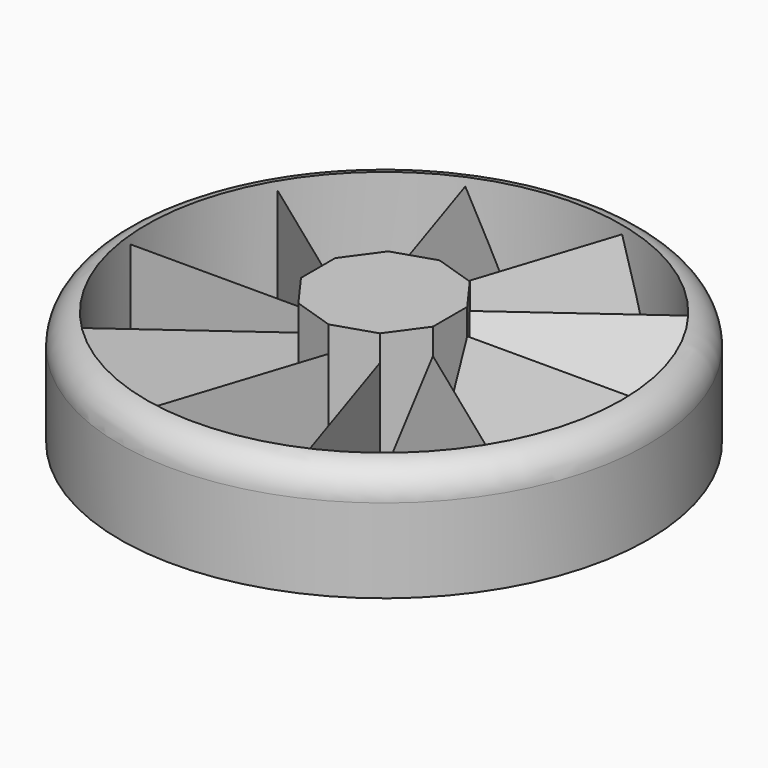
from build123d import *

# Parameters (mm, degrees)
F1_DEPTH  = 15
F3_DEPTH  = 20
F5_DEPTH  = 20
F14_DEPTH = 20
F15_DEPTH = 20
F16_DEPTH = 20
F17_DEPTH = 20
F18_DEPTH = 20
F19_DEPTH = 20
F20_DEPTH = 20
F21_DEPTH = 20
F23_R     = 30
F23_R_2   = 27
F24_DEPTH = 13
F26_R     = 1
F27_DEPTH = 8


# Not quite as in the source:
# - a fillet or chamfer that OpenCascade refuses, or shapes differently, is made with other operations: its cross-section is extruded or revolved along the edge and cut away or added


with BuildPart() as f1:
    # F0 (on Top) → F1 (new body)
    with BuildSketch(Plane.XY):
        Polygon((7.5, -2.4368977217), (7.5, 2.4368977217), (4.6352549156, 6.3798810626), (0, 7.8859666818), (-4.6352549156, 6.3798810626), (-7.5, 2.4368977217), (-7.5, -2.4368977217), (-4.6352549156, -6.3798810626), (0, -7.8859666818), (4.6352549156, -6.3798810626), align=None)
    extrude(amount=F1_DEPTH)

    # F2 (on face) → F3 (join)
    with BuildSketch(Plane(origin=(-2.3176274578, -7.1329238722, 0), x_dir=(0.9510565163, -0.3090169944, 0), z_dir=(-0.3090169944, -0.9510565163, 0))):
        Polygon((2.4368977217, 12.0518097386), (-2.4368977217, 0), (2.4368977217, 0), align=None)
    extrude(amount=F3_DEPTH)

    # F4 (on face) → F5 (join)
    with BuildSketch(Plane(origin=(-6.0676274578, -4.4083893922, 0), x_dir=(0.5877852523, -0.8090169944, 0), z_dir=(-0.8090169944, -0.5877852523, 0))):
        Polygon((2.4368977217, 12.0518097386), (-2.4368977217, 0), (2.4368977217, 0), align=None)
    extrude(amount=F5_DEPTH)

    # F13 (on face) → F14 (join)
    with BuildSketch(Plane(origin=(2.3176274578, -7.1329238722, 0), x_dir=(0.9510565163, 0.3090169944, 0), z_dir=(0.3090169944, -0.9510565163, 0))):
        Polygon((2.4368977217, 12.0518097386), (-2.4368977217, 0), (2.4368977217, 0), align=None)
    extrude(amount=F14_DEPTH)

    # F12 (on face) → F15 (join)
    with BuildSketch(Plane(origin=(6.0676274578, -4.4083893922, 0), x_dir=(0.5877852523, 0.8090169944, 0), z_dir=(0.8090169944, -0.5877852523, 0))):
        Polygon((2.4368977217, 12.0518097386), (-2.4368977217, 0), (2.4368977217, 0), align=None)
    extrude(amount=F15_DEPTH)

    # F11 (on face) → F16 (join)
    with BuildSketch(Plane.YZ.offset(7.5)):
        Polygon((2.4368977217, 12.0518097386), (-2.4368977217, 0), (2.4368977217, 0), align=None)
    extrude(amount=F16_DEPTH)

    # F10 (on face) → F17 (join)
    with BuildSketch(Plane(origin=(6.0676274578, 4.4083893922, 0), x_dir=(-0.5877852523, 0.8090169944, 0), z_dir=(0.8090169944, 0.5877852523, 0))):
        Polygon((2.4368977217, 12.0518097386), (-2.4368977217, 0), (2.4368977217, 0), align=None)
    extrude(amount=F17_DEPTH)

    # F9 (on face) → F18 (join)
    with BuildSketch(Plane(origin=(2.3176274578, 7.1329238722, 0), x_dir=(-0.9510565163, 0.3090169944, 0), z_dir=(0.3090169944, 0.9510565163, 0))):
        Polygon((2.4368977217, 12.0518097386), (-2.4368977217, 0), (2.4368977217, 0), align=None)
    extrude(amount=F18_DEPTH)

    # F8 (on face) → F19 (join)
    with BuildSketch(Plane(origin=(-2.3176274578, 7.1329238722, 0), x_dir=(-0.9510565163, -0.3090169944, 0), z_dir=(-0.3090169944, 0.9510565163, 0))):
        Polygon((2.4368977217, 12.0518097386), (-2.4368977217, 0), (2.4368977217, 0), align=None)
    extrude(amount=F19_DEPTH)

    # F7 (on face) → F20 (join)
    with BuildSketch(Plane(origin=(-6.0676274578, 4.4083893922, 0), x_dir=(-0.5877852523, -0.8090169944, 0), z_dir=(-0.8090169944, 0.5877852523, 0))):
        Polygon((2.4368977217, 12.0518097386), (-2.4368977217, 0), (2.4368977217, 0), align=None)
    extrude(amount=F20_DEPTH)

    # F6 (on face) → F21 (join)
    with BuildSketch(Plane(origin=(-7.5, 0, 0), x_dir=(0, -1, 0), z_dir=(-1, 0, 0))):
        Polygon((2.4368977217, 12.0518097386), (-2.4368977217, 0), (2.4368977217, 0), align=None)
    extrude(amount=F21_DEPTH)

    # F23 (on face) → F24 (join)
    with BuildSketch(Plane.XY):
        Circle(F23_R)
        Circle(F23_R_2, mode=Mode.SUBTRACT)
    extrude(amount=F24_DEPTH)

    # F25: fillet of radius 3.5 on 1 edges, made by hand

    # F25_s1 → F25_t2 (revolve, cut)
    with BuildSketch(Plane.XZ):
        with BuildLine():
            ThreePointArc((27, 13), (29.1457513111, 11.8271862323), (30, 9.5358983849))
            Line((30, 9.5358983849), (30, 13))
            Line((30, 13), (27, 13))
        make_face()
    revolve(axis=Axis((0, 0, 13), (0, 0, 1)), mode=Mode.SUBTRACT)

    # F26 (on face) → F27 (join)
    with BuildSketch(Plane.XY):
        Circle(F26_R)
    extrude(amount=F27_DEPTH)


solid = f1.part
